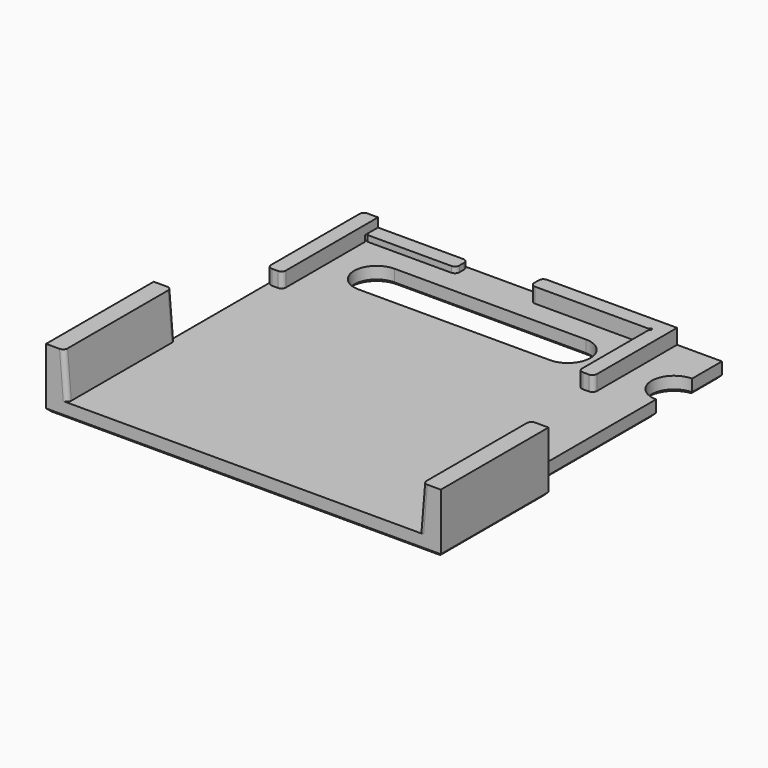
from build123d import *

# Parameters (mm, degrees)
F0_W      = 1.2
F0_H      = 9
F5_DEPTH  = 9
F7_DEPTH  = 1
F6_W      = 6
F6_H      = 1
F8_DEPTH  = 0.4
F9_DEPTH  = 1
F6_W_2    = 1
F6_H_2    = 1.2
F10_DEPTH = 1
F11_R     = 0.3
F13_DEPTH = 1
F14_DEPTH = 0.4
F15_SIZE  = 0.2


with BuildPart() as f2:
    # F2: sweep along a path in F1
    with BuildLine(Plane.XZ) as f2_path:
        Line((0, 0), (0, 1))
    # F0 (on Top) → F2 (sweep)
    with BuildSketch(Plane.XY):
        Polygon((-12, -8), (12, -8), (12, 1), (12, 8), (12, 9), (12, 17), (-12, 17), (-12, 9), (-12, 8), (-12, 1), align=None)
        with Locations((-12.6, -3.5)):
            Rectangle(F0_W, F0_H)
        with Locations((12.6, -3.5)):
            Rectangle(F0_W, F0_H)
    sweep(path=f2_path.line)

    # F3: sweep along a path in F1
    with BuildLine(Plane.XZ) as f3_path:
        Line((0, 0), (0, 1))
        Line((0, 1), (0, 4))
    # F0 (on Top) → F3 (sweep)
    with BuildSketch(Plane.XY):
        with Locations((-12.6, -3.5)):
            Rectangle(F0_W, F0_H)
        with Locations((12.6, -3.5)):
            Rectangle(F0_W, F0_H)
    sweep(path=f3_path.line)

    # F4 (on face) → F5 (join, through all)
    with BuildSketch(Plane.XZ.offset(8)):
        Polygon((-11.75, 1), (-12, 4), (-12, 1), align=None)
        Polygon((12, 1), (12, 4), (11.75, 1), align=None)
    extrude(amount=-F5_DEPTH)

    # F6 (on face) → F7 (join)
    with BuildSketch(Plane.XY.offset(1)):
        Polygon((-11, 17), (-12, 17), (-12, 15.8), (-12, 9), (-11, 9), (-11, 16), align=None)
        Polygon((9, 17), (0, 17), (0, 16), (8, 16), (8, 10), (9, 10), align=None)
    extrude(amount=F7_DEPTH)

    # F6 (on face) → F8 (join)
    with BuildSketch(Plane.XY.offset(1)):
        with Locations((-8, 16.5)):
            Rectangle(F6_W, F6_H)
    extrude(amount=F8_DEPTH)

    # F6 (on face) → F9 (cut, through all)
    with BuildSketch(Plane.XY.offset(1)):
        with BuildLine():
            ThreePointArc((-7.9, 14.5), (-9.4, 13), (-7.9, 11.5))
            Line((-7.9, 11.5), (4.9, 11.5))
            ThreePointArc((4.9, 11.5), (6.4, 13), (4.9, 14.5))
            Line((4.9, 14.5), (-7.9, 14.5))
        make_face()
        with BuildLine():
            Line((12, 11.5), (12, 14.5))
            ThreePointArc((12, 14.5), (10.5, 13), (12, 11.5))
        make_face()
    extrude(amount=-F9_DEPTH, mode=Mode.SUBTRACT)

    # F6 (on face) → F10 (join, through all)
    with BuildSketch(Plane.XY.offset(1)):
        with Locations((-12.5, 16.4)):
            Rectangle(F6_W_2, F6_H_2)
    extrude(amount=-F10_DEPTH)

    # F11
    f11_edges = [f2.edges().sort_by_distance(p)[0] for p in [
        (-11.875, -8, 2.5),
        (-11.875, 1, 2.5),
        (11.875, -8, 2.5),
        (-11, 9, 1.5),
        (0, 16, 1.5),
        (0, 17, 1.5),
        (8, 10, 1.5),
        (9, 10, 1.5),
        (-12, 9, 1.5),
        (-12, 17, 1.5),
        (-13, 17, 0.5),
        (-5, 16, 1.2),
        (-5, 17, 1.2),
        (11.875, 1, 2.5),
    ]]
    fillet(f11_edges, radius=F11_R)

    # F12 (on face) → F13 (cut, through all)
    with BuildSketch(Plane.XY.offset(1)):
        with BuildLine():
            ThreePointArc((8, 15.9), (8.0707106781, 15.9292893219), (8.1, 16))
            ThreePointArc((8.1, 16), (8, 16.1), (7.9, 16))
            Line((7.9, 16), (8, 16))
            Line((8, 16), (8, 15.9))
        make_face()
    extrude(amount=F13_DEPTH, mode=Mode.SUBTRACT)

    # F12 (on face) → F14 (cut, through all)
    with BuildSketch(Plane.XY.offset(1)):
        with BuildLine():
            Line((-11, 16), (-10.9, 16))
            ThreePointArc((-10.9, 16), (-11.0707106781, 16.0707106781), (-11, 15.9))
            Line((-11, 15.9), (-11, 16))
        make_face()
    extrude(amount=F14_DEPTH, mode=Mode.SUBTRACT)

    # F15
    f15_edges = [f2.edges().sort_by_distance(p)[0] for p in [
        (-0.35, 17, 0),
        (-12.912132, 16.912132, 0),
        (12, 15.75, 0),
        (-13, 16.25, 0),
        (10.5, 13, 0),
        (-12.5, 15.8, 0),
        (12, 6.25, 0),
        (-12, 8.4, 0),
        (12.6, 1, 0),
        (-12.6, 1, 0),
        (13.2, -3.5, 0),
        (-13.2, -3.5, 0),
        (0, -8, 0),
        (-9.4, 13, 0),
        (-1.5, 14.5, 0),
        (6.4, 13, 0),
        (-1.5, 11.5, 0),
    ]]
    chamfer(f15_edges, length=F15_SIZE)


solid = f2.part
